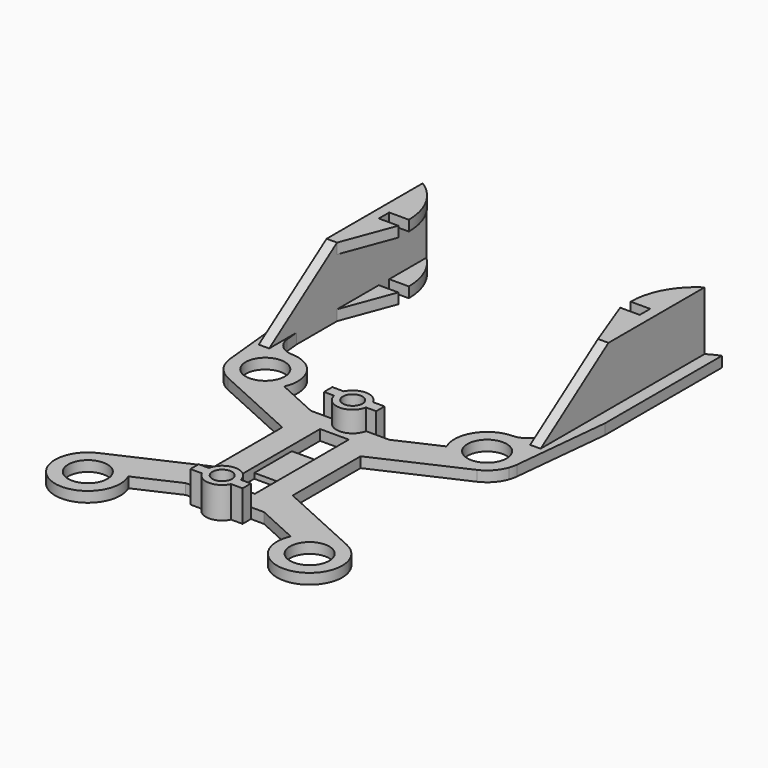
from build123d import *

# Parameters (mm, degrees)
F0_W          = 2.2
F0_H          = 3.6
F1_DEPTH      = 0.8
F0_R          = 0.75
F2_DEPTH      = 1.6
F2_DEPTH_BACK = 0.8
F3_DEPTH      = 0.4
F0_R_2        = 1.5
F4_DEPTH      = 0.8
F5_DEPTH      = 4.5
F5_DEPTH_BACK = 0.8
F6_W          = 1.5
F6_H          = 3.7
F6_H_2        = 2.6
F7_DEPTH      = 25
F7_DEPTH_BACK = 25
F9_DEPTH      = 0.8


# Not quite as in the source:
# - a feature of the source that left no trace in its solid (it failed there, or was rolled back) is left out
# - a pattern or mirror of a feature is missing from the dataset's text; its kind, count and spacing are read off the source's solid


with BuildPart() as f1:
    # F0 (on Top) → F1 (new body)
    with BuildSketch(Plane.XY):
        with BuildLine():
            Line((2, 7.6999996733), (1.2247448714, 7.6999996733))
            ThreePointArc((1.2247448714, 7.6999996733), (0, 6.6999996733), (-1.2247448714, 7.6999996733))
            Line((-1.2247448714, 7.6999996733), (-2, 7.6999996733))
            Line((-2, 7.6999996733), (-3, 7.6999996733))
            Line((-3, 7.6999996733), (-6.2240838063, 9.1654923125))
            ThreePointArc((-6.2240838063, 9.1654923125), (-7.622191396, 7.8591767294), (-9.5345073608, 7.9240834796))
            Line((-9.5345073608, 7.9240834796), (-3, 4.9538528611))
            Line((-3, 4.9538528611), (-3, -1.5538535145))
            Line((-3, -1.5538535145), (-9.5345073608, -4.5240841331))
            ThreePointArc((-9.5345073608, -4.5240841331), (-7.622191396, -4.4591773828), (-6.2240838063, -5.765492966))
            Line((-6.2240838063, -5.765492966), (-3, -4.3000003267))
            Line((-3, -4.3000003267), (-2, -4.3000003267))
            Line((-2, -4.3000003267), (-1.2247448714, -4.3000003267))
            ThreePointArc((-1.2247448714, -4.3000003267), (0, -3.3000003267), (1.2247448714, -4.3000003267))
            Line((1.2247448714, -4.3000003267), (2, -4.3000003267))
            Line((2, -4.3000003267), (3, -4.3000003267))
            Line((3, -4.3000003267), (6.2240838063, -5.765492966))
            ThreePointArc((6.2240838063, -5.765492966), (7.622191396, -4.4591773828), (9.5345073608, -4.5240841331))
            Line((9.5345073608, -4.5240841331), (3, -1.5538535145))
            Line((3, -1.5538535145), (3, 4.9538528611))
            Line((3, 4.9538528611), (9.5345073608, 7.9240834796))
            ThreePointArc((9.5345073608, 7.9240834796), (7.622191396, 7.8591767294), (6.2240838063, 9.1654923125))
            Line((6.2240838063, 9.1654923125), (3, 7.6999996733))
            Line((3, 7.6999996733), (2, 7.6999996733))
        make_face()
        Polygon((-1.1, 3.4999996733), (-1.1, 6.1999996733), (1.1, 6.1999996733), (1.1, 3.4999996733), (1.1, -0.1000003267), (1.1, -2.8000003267), (-1.1, -2.8000003267), (-1.1, -0.1000003267), align=None, mode=Mode.SUBTRACT)
        with Locations((0, 1.6999996733)):
            Rectangle(F0_W, F0_H)
    extrude(amount=-F1_DEPTH)

    # F0 (on Top) → F2 (join, two sides)
    with BuildSketch(Plane.XY) as f2_sk:
        with BuildLine():
            ThreePointArc((-1.2247448714, 7.6999996733), (-1.2399138495, 8.1084725282), (-1.122497216, 8.4999996733))
            Line((-1.122497216, 8.4999996733), (-2, 8.4999996733))
            Line((-2, 8.4999996733), (-2, 7.6999996733))
            Line((-2, 7.6999996733), (-1.2247448714, 7.6999996733))
        make_face()
        with BuildLine():
            ThreePointArc((1.2247448714, 7.6999996733), (1.2436701913, 7.8243634708), (1.25, 7.9499996733))
            ThreePointArc((1.25, 7.9499996733), (1.2177071733, 8.2322924999), (1.122497216, 8.4999996733))
            ThreePointArc((1.122497216, 8.4999996733), (0, 9.1999996733), (-1.122497216, 8.4999996733))
            ThreePointArc((-1.122497216, 8.4999996733), (-1.2399138495, 8.1084725282), (-1.2247448714, 7.6999996733))
            ThreePointArc((-1.2247448714, 7.6999996733), (0, 6.6999996733), (1.2247448714, 7.6999996733))
        make_face()
        with Locations((0, 7.9499996733)):
            Circle(F0_R, mode=Mode.SUBTRACT)
        with BuildLine():
            ThreePointArc((1.122497216, 8.4999996733), (1.2177071733, 8.2322924999), (1.25, 7.9499996733))
            ThreePointArc((1.25, 7.9499996733), (1.2436701913, 7.8243634708), (1.2247448714, 7.6999996733))
            Line((1.2247448714, 7.6999996733), (2, 7.6999996733))
            Line((2, 7.6999996733), (2, 8.4999996733))
            Line((2, 8.4999996733), (1.122497216, 8.4999996733))
        make_face()
        with BuildLine():
            Line((-1.2247448714, -4.3000003267), (-2, -4.3000003267))
            Line((-2, -4.3000003267), (-2, -5.1000003267))
            Line((-2, -5.1000003267), (-1.122497216, -5.1000003267))
            ThreePointArc((-1.122497216, -5.1000003267), (-1.2399138495, -4.7084731817), (-1.2247448714, -4.3000003267))
        make_face()
        with BuildLine():
            ThreePointArc((1.25, -4.5500003267), (1.2436701913, -4.4243641242), (1.2247448714, -4.3000003267))
            ThreePointArc((1.2247448714, -4.3000003267), (0, -3.3000003267), (-1.2247448714, -4.3000003267))
            ThreePointArc((-1.2247448714, -4.3000003267), (-1.2399138495, -4.7084731817), (-1.122497216, -5.1000003267))
            ThreePointArc((-1.122497216, -5.1000003267), (0, -5.8000003267), (1.122497216, -5.1000003267))
            ThreePointArc((1.122497216, -5.1000003267), (1.2177071733, -4.8322931534), (1.25, -4.5500003267))
        make_face()
        with Locations((0, -4.5500003267)):
            Circle(F0_R, mode=Mode.SUBTRACT)
        with BuildLine():
            Line((2, -5.1000003267), (2, -4.3000003267))
            Line((2, -4.3000003267), (1.2247448714, -4.3000003267))
            ThreePointArc((1.2247448714, -4.3000003267), (1.2436701913, -4.4243641242), (1.25, -4.5500003267))
            ThreePointArc((1.25, -4.5500003267), (1.2177071733, -4.8322931534), (1.122497216, -5.1000003267))
            Line((1.122497216, -5.1000003267), (2, -5.1000003267))
        make_face()
    extrude(amount=F2_DEPTH)
    extrude(f2_sk.sketch, amount=-F2_DEPTH_BACK)

    # F0 (on Top) → F3 (cut)
    with BuildSketch(Plane.XY):
        with Locations((0, 1.6999996733)):
            Rectangle(F0_W, F0_H)
    extrude(amount=-F3_DEPTH, mode=Mode.SUBTRACT)

    # F0 (on Top) → F4 (join)
    with BuildSketch(Plane.XY):
        with BuildLine():
            ThreePointArc((-9.5345073608, 7.9240834796), (-7.622191396, 7.8591767294), (-6.2240838063, 9.1654923125))
            ThreePointArc((-6.2240838063, 9.1654923125), (-6.3819707707, 11.5281382895), (-8.4399923541, 12.699279386))
            ThreePointArc((-8.4399923541, 12.699279386), (-10.3347684576, 11.8981235519), (-10.987178172, 9.9471266996))
            ThreePointArc((-10.987178172, 9.9471266996), (-10.9388236249, 9.6503276559), (-10.8551830715, 9.3614815161))
            ThreePointArc((-10.8551830715, 9.3614815161), (-10.3409314451, 8.5085590404), (-9.5345073608, 7.9240834796))
        make_face()
        with Locations((-8.5, 10.1999996733)):
            Circle(F0_R_2, mode=Mode.SUBTRACT)
        with BuildLine():
            ThreePointArc((8.4399923541, 12.699279386), (6.3819707707, 11.5281382895), (6.2240838063, 9.1654923125))
            ThreePointArc((6.2240838063, 9.1654923125), (7.622191396, 7.8591767294), (9.5345073608, 7.9240834796))
            ThreePointArc((9.5345073608, 7.9240834796), (10.3409314451, 8.5085590404), (10.8551830715, 9.3614815161))
            ThreePointArc((10.8551830715, 9.3614815161), (10.9388236249, 9.6503276559), (10.987178172, 9.9471266996))
            ThreePointArc((10.987178172, 9.9471266996), (10.3347684576, 11.8981235519), (8.4399923541, 12.699279386))
        make_face()
        with Locations((8.5, 10.1999996733)):
            Circle(F0_R_2, mode=Mode.SUBTRACT)
        with BuildLine():
            ThreePointArc((-6.2240838063, -5.765492966), (-7.622191396, -4.4591773828), (-9.5345073608, -4.5240841331))
            ThreePointArc((-9.5345073608, -4.5240841331), (-10.3409314451, -5.1085596938), (-10.8551830715, -5.9614821695))
            ThreePointArc((-10.8551830715, -5.9614821695), (-8.394294033, -9.2977645767), (-6.2240838063, -5.765492966))
        make_face()
        with Locations((-8.5, -6.8000003267)):
            Circle(F0_R_2, mode=Mode.SUBTRACT)
        with BuildLine():
            ThreePointArc((10.8551830715, -5.9614821695), (10.3409314451, -5.1085596938), (9.5345073608, -4.5240841331))
            ThreePointArc((9.5345073608, -4.5240841331), (7.622191396, -4.4591773828), (6.2240838063, -5.765492966))
            ThreePointArc((6.2240838063, -5.765492966), (8.394294033, -9.2977645767), (10.8551830715, -5.9614821695))
        make_face()
        with Locations((8.5, -6.8000003267)):
            Circle(F0_R_2, mode=Mode.SUBTRACT)
        with BuildLine():
            ThreePointArc((-10.987178172, 9.9471266996), (-10.3347684576, 11.8981235519), (-8.4399923541, 12.699279386))
            ThreePointArc((-8.4399923541, 12.699279386), (-9.4228620937, 13.0979861391), (-9.8962946697, 14.0471234295))
            Line((-9.8962946697, 14.0471234295), (-10, 15.0671360866))
            Line((-10, 15.0671360866), (-10, 18.9499996733))
            Line((-10, 18.9499996733), (-10.8, 18.9499996733))
            Line((-10.8, 18.9499996733), (-10.8, 28.1583247558))
            ThreePointArc((-10.8, 28.1583247558), (-11.2623378592, 28.4213381914), (-11.75, 28.6337481721))
            Line((-11.75, 28.6337481721), (-11.75, 17.4499996733))
            Line((-11.75, 17.4499996733), (-10.987178172, 9.9471266996))
        make_face()
        with BuildLine():
            ThreePointArc((9.8962946697, 14.0471234295), (9.4228620937, 13.0979861391), (8.4399923541, 12.699279386))
            ThreePointArc((8.4399923541, 12.699279386), (10.3347684576, 11.8981235519), (10.987178172, 9.9471266996))
            Line((10.987178172, 9.9471266996), (11.75, 17.4499996733))
            Line((11.75, 17.4499996733), (11.75, 28.6337481721))
            ThreePointArc((11.75, 28.6337481721), (11.2623378592, 28.4213381914), (10.8, 28.1583247558))
            Line((10.8, 28.1583247558), (10.8, 18.9499996733))
            Line((10.8, 18.9499996733), (10, 18.9499996733))
            Line((10, 18.9499996733), (10, 15.0671360866))
            Line((10, 15.0671360866), (9.8962946697, 14.0471234295))
        make_face()
    extrude(amount=-F4_DEPTH)

    # F0 (on Top) → F5 (join, two sides)
    with BuildSketch(Plane.XY) as f5_sk:
        with BuildLine():
            Line((-10.8, 18.9499996733), (-10, 18.9499996733))
            Line((-10, 18.9499996733), (-10, 22.9499996733))
            Line((-10, 22.9499996733), (-10, 23.9499996733))
            Line((-10, 23.9499996733), (-10, 27.5207138876))
            ThreePointArc((-10, 27.5207138876), (-10.383650067, 27.860033317), (-10.8, 28.1583247558))
            Line((-10.8, 28.1583247558), (-10.8, 18.9499996733))
        make_face()
        Polygon((-10, 22.9499996733), (-10, 18.9499996733), (-8.5, 22.9499996733), align=None)
        with BuildLine():
            ThreePointArc((-8.5, 23.9499996733), (-8.8902277714, 25.8864913464), (-10, 27.5207138876))
            Line((-10, 27.5207138876), (-10, 23.9499996733))
            Line((-10, 23.9499996733), (-8.5, 23.9499996733))
        make_face()
        with BuildLine():
            Line((10, 22.9499996733), (10, 18.9499996733))
            Line((10, 18.9499996733), (10.8, 18.9499996733))
            Line((10.8, 18.9499996733), (10.8, 28.1583247558))
            ThreePointArc((10.8, 28.1583247558), (10.383650067, 27.860033317), (10, 27.5207138876))
            Line((10, 27.5207138876), (10, 23.9499996733))
            Line((10, 23.9499996733), (10, 22.9499996733))
        make_face()
        Polygon((8.5, 22.9499996733), (10, 18.9499996733), (10, 22.9499996733), align=None)
        with BuildLine():
            Line((10, 23.9499996733), (10, 27.5207138876))
            ThreePointArc((10, 27.5207138876), (8.8902277714, 25.8864913464), (8.5, 23.9499996733))
            Line((8.5, 23.9499996733), (10, 23.9499996733))
        make_face()
    extrude(amount=F5_DEPTH)
    extrude(f5_sk.sketch, amount=-F5_DEPTH_BACK)

    # F6 (on face) → F7 (cut, two sides)
    with BuildSketch(Plane(origin=(0, 22.9499996733, 0), x_dir=(-1, 0, 0), z_dir=(0, 1, 0))) as f7_sk:
        with Locations((9.25, 1.85)):
            Rectangle(F6_W, F6_H)
        with Locations((-9.25, 1.85)):
            Rectangle(F6_W, F6_H_2)
    extrude(amount=-F7_DEPTH, mode=Mode.SUBTRACT)
    extrude(f7_sk.sketch, amount=F7_DEPTH_BACK, mode=Mode.SUBTRACT)

    # F8 (on face) → F9 (join)
    with BuildSketch(Plane(origin=(10, 0, 0), x_dir=(0, -1, 0), z_dir=(-1, 0, 0))):
        Polygon((-12.4499996733, 0), (-18.9499996733, 4.5), (-18.9499996733, 0), align=None)
    f9 = extrude(amount=-F9_DEPTH)

    # F9_copies: F9 across plane
    add(f9.mirror(Plane(origin=(0, 0, 0), x_dir=(0, 0, -1), z_dir=(-1, 0, 0))))


solid = f1.part
